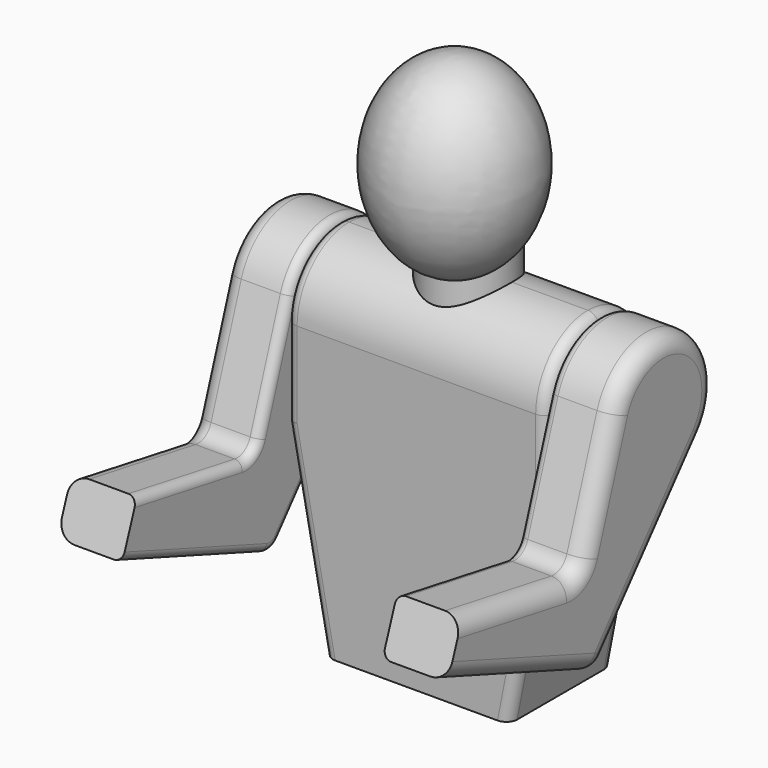
from build123d import *

# Parameters (mm, degrees)
F1_DEPTH    = 19.05
F2_T1_DEPTH = 171.45
F3_W        = 12.7
F3_H        = 38.1
F7_R        = 3.175
F8_R        = 3.175
F10_DEPTH   = 19.05
F11_R       = 5.08
F11_2_R     = 5.08
F14_R       = 2.54
F14_2_R     = 2.54


# Not quite as in the source:
# - a fillet or chamfer that OpenCascade refuses, or shapes differently, is made with other operations: its cross-section is extruded or revolved along the edge and cut away or added
# - two fillets or chamfers of one size are made in one step
# - a pattern or mirror of a feature is missing from the dataset's text; its kind, count and spacing are read off the source's solid


with BuildPart() as f1:
    # F0 (on Front) → F1 (new body, symmetric)
    with BuildSketch(Plane.XZ):
        Polygon((-38.1, 57.15), (-26.9875, 0), (26.9875, 0), (38.1, 57.15), (38.1, 101.6), (-38.1, 101.6), align=None)
    extrude(amount=F1_DEPTH, both=True)

    # F2: fillet of radius 19.05 on 2 edges, made by hand

    # F2_s2 → F2_t1 (cut)
    with BuildSketch(Plane.YZ.offset(-85.725)):
        with BuildLine():
            ThreePointArc((0, 101.6), (-13.4703841816, 96.0203841816), (-19.05, 82.55))
            Line((-19.05, 82.55), (-19.05, 101.6))
            Line((-19.05, 101.6), (0, 101.6))
        make_face()
        with BuildLine():
            ThreePointArc((0, 101.6), (13.4703841816, 96.0203841816), (19.05, 82.55))
            Line((19.05, 82.55), (19.05, 101.6))
            Line((19.05, 101.6), (0, 101.6))
        make_face()
    extrude(amount=F2_T1_DEPTH, mode=Mode.SUBTRACT)

    # F3 (on Front) → F4 (revolve)
    with BuildSketch(Plane.XZ):
        with Locations((6.35, 101.6)):
            Rectangle(F3_W, F3_H)
    revolve(axis=Axis((0, 0, 41.275), (0, 0, -1)))

    # F5 (on Right) → F6 (revolve)
    with BuildSketch(Plane.YZ):
        with BuildLine():
            Line((-5.08, 158.115), (-5.08, 102.235))
            add(Edge.make_bspline(
                [(-5.08, 102.235), (17.145, 102.235), (17.145, 130.175), (17.145, 158.115), (-5.08, 158.115)],
                knots=[3.1415926536, 3.1415926536, 3.1415926536, 4.7123889804, 4.7123889804, 6.2831853072, 6.2831853072, 6.2831853072], degree=2, weights=[1, 0.7071067812, 1, 0.7071067812, 1]))
        make_face()
    revolve(axis=Axis((0, -5.08, 55.275326029), (0, 0, -1)))

    # F7
    f7_edges = [f1.edges().sort_by_distance(p)[0] for p in [
        (-38.1, 0, 57.15),
        (38.1, 0, 57.15),
    ]]
    fillet(f7_edges, radius=F7_R)

    # F8
    f8_edges = [f1.edges().sort_by_distance(p)[0] for p in [
        (32.514564, -19.05, 28.424903),
        (-32.514564, -19.05, 28.424903),
        (-32.514564, 19.05, 28.424903),
        (-38.1, 19.05, 70.002908),
        (-38.085374, 19.05, 57.151409),
        (38.1, 19.05, 70.002908),
        (38.085374, 19.05, 57.151409),
        (32.514564, 19.05, 28.424903),
        (-38.085374, -19.05, 57.151409),
        (38.085374, -19.05, 57.151409),
        (-38.1, -13.470384, 96.020384),
        (-38.1, 13.470384, 96.020384),
        (38.1, 13.470384, 96.020384),
        (38.1, -13.470384, 96.020384),
    ]]
    fillet(f8_edges, radius=F8_R)


with BuildPart() as f10:
    # F9 (on face) → F10 (new body)
    with BuildSketch(Plane.YZ.offset(38.1)):
        with BuildLine():
            Line((-23.622, 24.761857734), (14.5931466414, 70.3048960355))
            ThreePointArc((14.5931466414, 70.3048960355), (9.3486979196, 99.1483236264), (-18.0359002739, 88.6826015123))
            Line((-18.0359002739, 88.6826015123), (-30.48, 52.084668122))
            Line((-30.48, 52.084668122), (-73.66, 59.698467149))
            Line((-73.66, 59.698467149), (-79.0350757506, 44.9305678964))
            Line((-79.0350757506, 44.9305678964), (-23.622, 24.761857734))
        make_face()
    extrude(amount=F10_DEPTH)


with BuildPart() as f10_copies_1:
    # F10_copies: instance of F10
    add(f10.part.mirror(Plane(origin=(0, 0, 0), x_dir=(0, 0, -1), z_dir=(-1, 0, 0))))

    # F11#2
    f11_2_edges = [f10_copies_1.edges().sort_by_distance(p)[0] for p in [
        (-47.625, -23.622, 24.761858),
        (-57.15, -51.328538, 34.846213),
        (-57.15, -4.514427, 47.533377),
        (-57.15, 9.348698, 99.148324),
        (-47.625, -30.48, 52.084668),
        (-57.15, -24.25795, 70.383635),
        (-57.15, -52.07, 55.891568),
    ]]
    fillet(f11_2_edges, radius=F11_2_R)

    # F14#2
    f14_2_edges = [f10_copies_1.edges().sort_by_distance(p)[0] for p in [
        (-38.1, -52.999807, 35.454505),
        (-38.1, -23.912275, 25.845177),
        (-38.1, -54.214758, 56.269746),
        (-38.1, 9.348698, 99.148324),
        (-38.1, -31.300658, 53.47175),
        (-38.1, -23.556855, 72.445545),
    ]]
    fillet(f14_2_edges, radius=F14_2_R)


with BuildPart() as f10_1:
    add(f10.part)

    # F11
    f11_edges = [f10_1.edges().sort_by_distance(p)[0] for p in [
        (47.625, -30.48, 52.084668),
        (47.625, -23.622, 24.761858),
        (57.15, -51.328538, 34.846213),
        (57.15, -4.514427, 47.533377),
        (57.15, 9.348698, 99.148324),
        (57.15, -24.25795, 70.383635),
        (57.15, -52.07, 55.891568),
    ]]
    fillet(f11_edges, radius=F11_R)

    # F14
    f14_edges = [f10_1.edges().sort_by_distance(p)[0] for p in [
        (38.1, -3.371211, 48.895808),
        (38.1, -52.999807, 35.454505),
        (38.1, -23.912275, 25.845177),
        (38.1, -54.214758, 56.269746),
        (38.1, 9.348698, 99.148324),
        (38.1, -31.300658, 53.47175),
        (38.1, -23.556855, 72.445545),
    ]]
    fillet(f14_edges, radius=F14_R)


solid = Compound([f1.part, f10_copies_1.part, f10_1.part])
